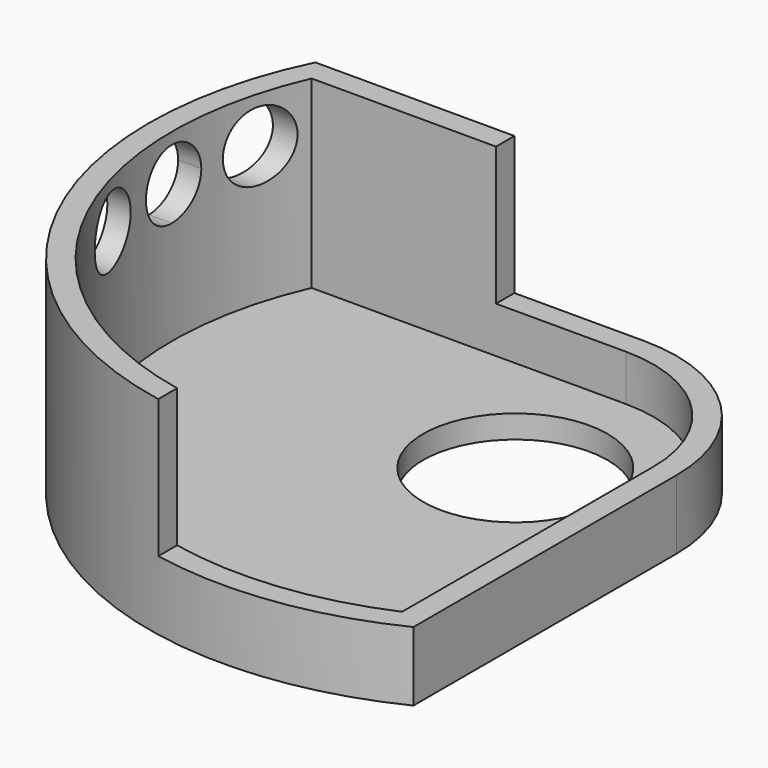
from build123d import *

# Parameters (mm, degrees)
F0_R          = 2
F1_DEPTH      = 0.5
F2_DEPTH      = 1.5
F3_DEPTH      = 4.5
F5_R          = 0.75
F6_DEPTH      = 22
F6_DEPTH_BACK = 1.8118981114


# Not quite as in the source:
# - an extrude ends at something that could not be found from the text; its depth is read off the source's solid
# - a feature names something its author has since deleted; it is built from what else it names


with BuildPart() as f1:
    # F0 (on Top) → F1 (new body)
    with BuildSketch(Plane.XY):
        with BuildLine():
            ThreePointArc((3, -1.8027756377), (3.3726843908, -0.9354143467), (3.5, 0))
            ThreePointArc((3.5, 0), (2.4748737342, 2.4748737342), (0, 3.5))
            ThreePointArc((0, 3.5), (-0.9354143467, 3.3726843908), (-1.8027756377, 3))
            Line((-1.8027756377, 3), (0, 3))
            ThreePointArc((0, 3), (2.1213203436, 2.1213203436), (3, 0))
            Line((3, 0), (3, -1.8027756377))
        make_face()
        with BuildLine():
            ThreePointArc((-1.8027756377, 3), (-0.9354143467, 3.3726843908), (0, 3.5))
            Line((0, 3.5), (-2.8192741549, 3.5))
            Line((-2.8192741549, 3.5), (-2.8192741549, 3))
            Line((-2.8192741549, 3), (-1.8027756377, 3))
        make_face()
        with BuildLine():
            Line((3.5, -7.1381019886), (3.5, -6.5766632877))
            ThreePointArc((3.5, -6.5766632877), (3.2522630595, -6.7026326911), (3, -6.8192741549))
            ThreePointArc((3, -6.8192741549), (0.7871839081, -7.4082954514), (-1.5, -7.2974310548))
            Line((-1.5, -7.2974310548), (-1.5, -7.8072082078))
            ThreePointArc((-1.5, -7.8072082078), (1.0544789155, -7.8797572435), (3.5, -7.1381019886))
        make_face()
        with BuildLine():
            Line((3.5, -6.5766632877), (3.5, 0))
            ThreePointArc((3.5, 0), (3.3726843908, -0.9354143467), (3, -1.8027756377))
            Line((3, -1.8027756377), (3, -6.8192741549))
            ThreePointArc((3, -6.8192741549), (3.2522630595, -6.7026326911), (3.5, -6.5766632877))
        make_face()
        with BuildLine():
            Line((3, -6.8192741549), (3, -1.8027756377))
            ThreePointArc((3, -1.8027756377), (-2.4748737342, -2.4748737342), (-1.8027756377, 3))
            Line((-1.8027756377, 3), (-2.8192741549, 3))
            Line((-2.8192741549, 3), (-6.8192741549, 3))
            ThreePointArc((-6.8192741549, 3), (-6.619052213, -3.4191589319), (-1.5, -7.2974310548))
            ThreePointArc((-1.5, -7.2974310548), (0.7871839081, -7.4082954514), (3, -6.8192741549))
        make_face()
        with BuildLine():
            ThreePointArc((-1.8027756377, 3), (-2.4748737342, -2.4748737342), (3, -1.8027756377))
            Line((3, -1.8027756377), (3, 0))
            ThreePointArc((3, 0), (-2.1213203436, -2.1213203436), (0, 3))
            Line((0, 3), (-1.8027756377, 3))
        make_face()
        with BuildLine():
            ThreePointArc((0, 3), (-2.1213203436, -2.1213203436), (3, 0))
            ThreePointArc((3, 0), (2.1213203436, 2.1213203436), (0, 3))
        make_face()
        Circle(F0_R, mode=Mode.SUBTRACT)
    extrude(amount=F1_DEPTH)

    # F0 (on Top) → F2 (join)
    with BuildSketch(Plane.XY):
        with BuildLine():
            Line((3.5, -7.1381019886), (3.5, -6.5766632877))
            ThreePointArc((3.5, -6.5766632877), (3.2522630595, -6.7026326911), (3, -6.8192741549))
            ThreePointArc((3, -6.8192741549), (0.7871839081, -7.4082954514), (-1.5, -7.2974310548))
            Line((-1.5, -7.2974310548), (-1.5, -7.8072082078))
            ThreePointArc((-1.5, -7.8072082078), (1.0544789155, -7.8797572435), (3.5, -7.1381019886))
        make_face()
        with BuildLine():
            Line((3.5, -6.5766632877), (3.5, 0))
            ThreePointArc((3.5, 0), (3.3726843908, -0.9354143467), (3, -1.8027756377))
            Line((3, -1.8027756377), (3, -6.8192741549))
            ThreePointArc((3, -6.8192741549), (3.2522630595, -6.7026326911), (3.5, -6.5766632877))
        make_face()
        with BuildLine():
            ThreePointArc((3, -1.8027756377), (3.3726843908, -0.9354143467), (3.5, 0))
            ThreePointArc((3.5, 0), (2.4748737342, 2.4748737342), (0, 3.5))
            ThreePointArc((0, 3.5), (-0.9354143467, 3.3726843908), (-1.8027756377, 3))
            Line((-1.8027756377, 3), (0, 3))
            ThreePointArc((0, 3), (2.1213203436, 2.1213203436), (3, 0))
            Line((3, 0), (3, -1.8027756377))
        make_face()
        with BuildLine():
            ThreePointArc((-1.8027756377, 3), (-0.9354143467, 3.3726843908), (0, 3.5))
            Line((0, 3.5), (-2.8192741549, 3.5))
            Line((-2.8192741549, 3.5), (-2.8192741549, 3))
            Line((-2.8192741549, 3), (-1.8027756377, 3))
        make_face()
        with BuildLine():
            Line((-2.8192741549, 3), (-2.8192741549, 3.5))
            Line((-2.8192741549, 3.5), (-6.5766632877, 3.5))
            ThreePointArc((-6.5766632877, 3.5), (-6.7026326911, 3.2522630595), (-6.8192741549, 3))
            Line((-6.8192741549, 3), (-2.8192741549, 3))
        make_face()
        with BuildLine():
            ThreePointArc((-6.8192741549, 3), (-6.7026326911, 3.2522630595), (-6.5766632877, 3.5))
            Line((-6.5766632877, 3.5), (-7.1381019886, 3.5))
            ThreePointArc((-7.1381019886, 3.5), (-7.114593513, -3.5475426911), (-1.5, -7.8072082078))
            Line((-1.5, -7.8072082078), (-1.5, -7.2974310548))
            ThreePointArc((-1.5, -7.2974310548), (-6.619052213, -3.4191589319), (-6.8192741549, 3))
        make_face()
    extrude(amount=F2_DEPTH)

    # F0 (on Top) → F3 (join)
    with BuildSketch(Plane.XY):
        with BuildLine():
            ThreePointArc((-6.8192741549, 3), (-6.7026326911, 3.2522630595), (-6.5766632877, 3.5))
            Line((-6.5766632877, 3.5), (-7.1381019886, 3.5))
            ThreePointArc((-7.1381019886, 3.5), (-7.114593513, -3.5475426911), (-1.5, -7.8072082078))
            Line((-1.5, -7.8072082078), (-1.5, -7.2974310548))
            ThreePointArc((-1.5, -7.2974310548), (-6.619052213, -3.4191589319), (-6.8192741549, 3))
        make_face()
        with BuildLine():
            Line((-2.8192741549, 3), (-2.8192741549, 3.5))
            Line((-2.8192741549, 3.5), (-6.5766632877, 3.5))
            ThreePointArc((-6.5766632877, 3.5), (-6.7026326911, 3.2522630595), (-6.8192741549, 3))
            Line((-6.8192741549, 3), (-2.8192741549, 3))
        make_face()
    extrude(amount=F3_DEPTH)

    # F5 (on plane+point) → F6 (cut, two sides)
    with BuildSketch(Plane.YZ.offset(-7.1381019886)) as f6_sk:
        with BuildLine():
            ThreePointArc((2.75, 3.5), (2, 4.25), (1.25, 3.5))
            ThreePointArc((1.25, 3.5), (2, 2.75), (2.75, 3.5))
        make_face()
        with BuildLine():
            Line((0, 3.5), (0, 2.75))
            ThreePointArc((0, 2.75), (0.5303300859, 2.9696699141), (0.75, 3.5))
            Line((0.75, 3.5), (0, 3.5))
        make_face()
        with BuildLine():
            Line((-0.75, 3.5), (0, 3.5))
            Line((0, 3.5), (0.75, 3.5))
            ThreePointArc((0.75, 3.5), (0, 4.25), (-0.75, 3.5))
        make_face()
        with BuildLine():
            ThreePointArc((-0.75, 3.5), (-0.5303300859, 2.9696699141), (0, 2.75))
            Line((0, 2.75), (0, 3.5))
            Line((0, 3.5), (-0.75, 3.5))
        make_face()
        with Locations((-2, 3.5)):
            Circle(F5_R)
    extrude(amount=F6_DEPTH, mode=Mode.SUBTRACT)
    extrude(f6_sk.sketch, amount=-F6_DEPTH_BACK, mode=Mode.SUBTRACT)


solid = f1.part
